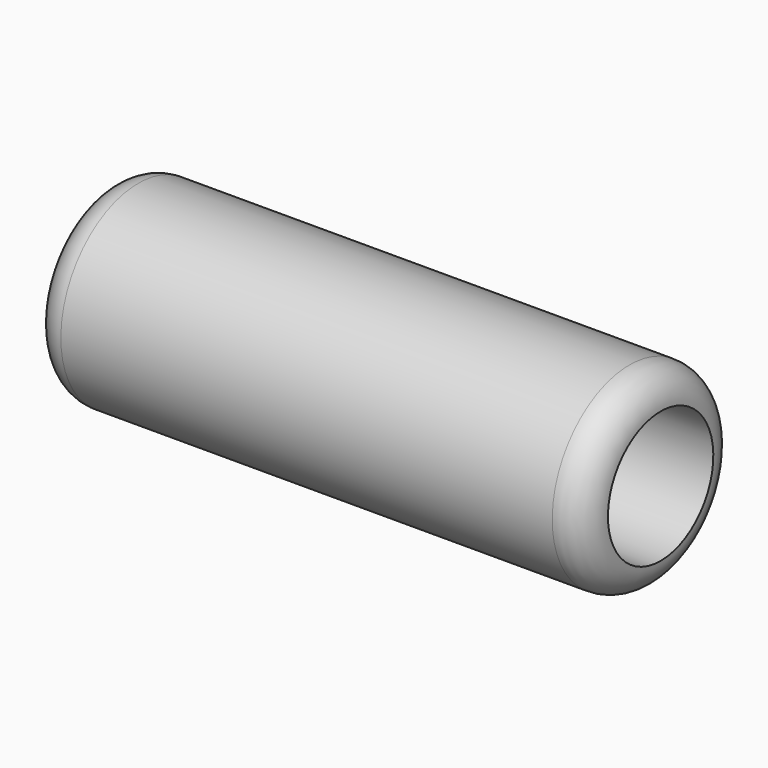
from build123d import *

# Parameters (mm, degrees)
F2_R = 6.34999


# Not quite as in the source:
# - a fillet or chamfer is up to 0.001 mm smaller than in the source, because OpenCascade refuses the exact size


with BuildPart() as f1:
    # F0 (on Front) → F1 (revolve)
    with BuildSketch(Plane.XZ):
        Polygon((-51.2101510014, -25.1150900284), (-55.1725510014, -25.1150900284), (-55.1725510014, -42.5902900284), (58.3400489986, -42.5902900284), (58.3400489986, -36.2402900284), (-51.2101510014, -36.2402900284), align=None)
    revolve(axis=Axis((-5.4417531937, 0, -22.7274900284), (1, 0, 0)))

    # F2 (radius 6.35 in the source; OpenCascade refuses exactly that, so slightly less here)
    f2_edges = [f1.edges().sort_by_distance(p)[0] for p in [
        (-55.172551, 0, -2.86469),
        (58.340049, 0, -2.86469),
    ]]
    fillet(f2_edges, radius=F2_R)


solid = f1.part
